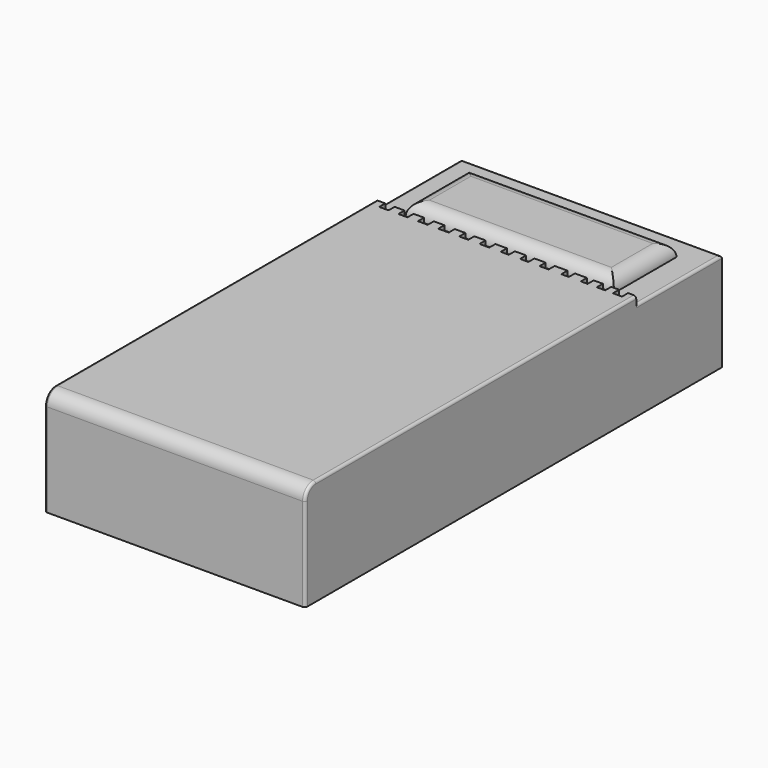
from build123d import *

# Parameters (mm, degrees)
F0_W         = 100
F0_H         = 37.7952754252
F1_DEPTH     = 200
F2_W         = 80
F2_H         = 30
F3_DEPTH     = 5
F4_T4_DEPTH  = 55.4
F4_T9_DEPTH  = 105.4
F4_T14_DEPTH = 55.4
F4_T19_DEPTH = 105.4
F5_W         = 100
F5_H         = 155.959841609
F6_DEPTH     = 3
F7_W         = 18.5192480683
F7_H         = 2.9272809625
F7_W_2       = 4.0360428393
F7_W_3       = 4.3243318796
F7_W_4       = 4.4076992199
F7_W_5       = 4.324331414
F7_W_6       = 4.9009080976
F7_W_7       = 4.6126190573
F7_W_8       = 16.3274921477
F8_DEPTH     = 3
F9_W         = 3.4559369087
F9_H         = 2.9272809625
F9_W_2       = 3.5711340606
F9_W_3       = 3.2255388796
F10_DEPTH    = 3
F11_R        = 5.08
F12_R        = 1


# Not quite as in the source:
# - a fillet or chamfer that OpenCascade refuses, or shapes differently, is made with other operations: its cross-section is extruded or revolved along the edge and cut away or added


with BuildPart() as f1:
    # F0 (on Front) → F1 (new body)
    with BuildSketch(Plane.XZ):
        with Locations((-0.3143809736, 22.1638707444)):
            Rectangle(F0_W, F0_H)
    extrude(amount=F1_DEPTH)

    # F2 (on face) → F3 (join)
    with BuildSketch(Plane.XY.offset(41.061508457)):
        with Locations((-0.3143809736, -24.2907730862)):
            Rectangle(F2_W, F2_H)
    extrude(amount=F3_DEPTH)

    # F4: fillet of radius 5.08 on 4 edges, made by hand


with BuildPart() as f4_tool2:
    # F4_s3 → F4_t4 (new body)
    with BuildSketch(Plane.XZ.offset(51.9907730862)):
        with BuildLine():
            ThreePointArc((39.6856190264, 40.981508457), (38.1977214749, 44.5736109055), (34.6056190264, 46.061508457))
            Line((34.6056190264, 46.061508457), (39.6856190264, 46.061508457))
            Line((39.6856190264, 46.061508457), (39.6856190264, 40.981508457))
        make_face()
    extrude(amount=-F4_T4_DEPTH)

    split(bisect_by=Plane.XY.offset(41.061508457), keep=Keep.TOP)


with BuildPart() as f1_1:
    add(f1.part)

    # F4_t1: cut F4_tool2
    add(f4_tool2.part, mode=Mode.SUBTRACT)


with BuildPart() as f4_tool7:
    # F4_s8 → F4_t9 (new body)
    with BuildSketch(Plane.YZ.offset(52.3856190264)):
        with BuildLine():
            ThreePointArc((-9.2907730862, 40.981508457), (-10.7786706378, 44.5736109055), (-14.3707730862, 46.061508457))
            Line((-14.3707730862, 46.061508457), (-9.2907730862, 46.061508457))
            Line((-9.2907730862, 46.061508457), (-9.2907730862, 40.981508457))
        make_face()
    extrude(amount=-F4_T9_DEPTH)

    split(bisect_by=Plane.XY.offset(41.061508457), keep=Keep.TOP)


with BuildPart() as f1_2:
    add(f1_1.part)

    # F4_t6: cut F4_tool7
    add(f4_tool7.part, mode=Mode.SUBTRACT)


with BuildPart() as f4_tool12:
    # F4_s13 → F4_t14 (new body)
    with BuildSketch(Plane.XZ.offset(-3.4092269138)):
        with BuildLine():
            ThreePointArc((-40.3143809736, 40.981508457), (-38.826483422, 44.5736109055), (-35.2343809736, 46.061508457))
            Line((-35.2343809736, 46.061508457), (-40.3143809736, 46.061508457))
            Line((-40.3143809736, 46.061508457), (-40.3143809736, 40.981508457))
        make_face()
    extrude(amount=F4_T14_DEPTH)

    split(bisect_by=Plane.XY.offset(41.061508457), keep=Keep.TOP)


with BuildPart() as f1_3:
    add(f1_2.part)

    # F4_t11: cut F4_tool12
    add(f4_tool12.part, mode=Mode.SUBTRACT)


with BuildPart() as f4_tool17:
    # F4_s18 → F4_t19 (new body)
    with BuildSketch(Plane.YZ.offset(-53.0143809736)):
        with BuildLine():
            ThreePointArc((-39.2907730862, 40.981508457), (-37.8028755347, 44.5736109055), (-34.2107730862, 46.061508457))
            Line((-34.2107730862, 46.061508457), (-39.2907730862, 46.061508457))
            Line((-39.2907730862, 46.061508457), (-39.2907730862, 40.981508457))
        make_face()
    extrude(amount=F4_T19_DEPTH)

    split(bisect_by=Plane.XY.offset(41.061508457), keep=Keep.TOP)


with BuildPart() as f1_4:
    add(f1_3.part)

    # F4_t16: cut F4_tool17
    add(f4_tool17.part, mode=Mode.SUBTRACT)

    # F5 (on face) → F6 (join)
    with BuildSketch(Plane.XY.offset(41.061508457)):
        with Locations((-0.3143809736, -122.0200791955)):
            Rectangle(F5_W, F5_H)
    extrude(amount=F6_DEPTH)

    # F7 (on face) → F8 (join)
    with BuildSketch(Plane.XY.offset(41.061508457)):
        with Locations((-41.0547569394, -42.5765179098)):
            Rectangle(F7_W, F7_H)
        with Locations((-26.0293576866, -42.5765179098)):
            Rectangle(F7_W_2, F7_H)
        with Locations((-17.9572720081, -42.5765179098)):
            Rectangle(F7_W_2, F7_H)
        with Locations((-10.31761989, -42.5765179098)):
            Rectangle(F7_W_3, F7_H)
        with Locations((-2.2038496099, -42.5765179098)):
            Rectangle(F7_W_4, F7_H)
        with Locations((5.2499750163, -42.5765179098)):
            Rectangle(F7_W_5, F7_H)
        with Locations((12.7454819158, -42.5765179098)):
            Rectangle(F7_W_3, F7_H)
        with Locations((20.817569457, -42.5765179098)):
            Rectangle(F7_W_6, F7_H)
        with Locations((28.4572215751, -42.5765179098)):
            Rectangle(F7_W_7, F7_H)
        with Locations((41.5218729526, -42.5765179098)):
            Rectangle(F7_W_8, F7_H)
    extrude(amount=F8_DEPTH)

    # F9 (on face) → F10 (cut)
    with BuildSketch(Plane.XY.offset(44.061508457)):
        with Locations((-37.5542342663, -42.5765179098)):
            Rectangle(F9_W, F9_H)
        with Locations((-44.8692981154, -42.5765179098)):
            Rectangle(F9_W_2, F9_H)
        with Locations((38.4763423353, -42.5765179098)):
            Rectangle(F9_W_3, F9_H)
        with Locations((44.8122248054, -42.5765179098)):
            Rectangle(F9_W, F9_H)
    extrude(amount=-F10_DEPTH, mode=Mode.SUBTRACT)

    # F11
    f11_edges = [f1_4.edges().sort_by_distance(p)[0] for p in [
        (-0.314381, -200, 44.061508),
    ]]
    fillet(f11_edges, radius=F11_R)

    # F12
    f12_edges = [f1_4.edges().sort_by_distance(p)[0] for p in [
        (49.685619, -20.556439, 41.061508),
        (-0.314381, 0, 41.061508),
        (-50.314381, -20.556439, 41.061508),
        (-50.314381, -118.016439, 44.061508),
        (49.685619, -118.016439, 44.061508),
    ]]
    fillet(f12_edges, radius=F12_R)


solid = f1_4.part
